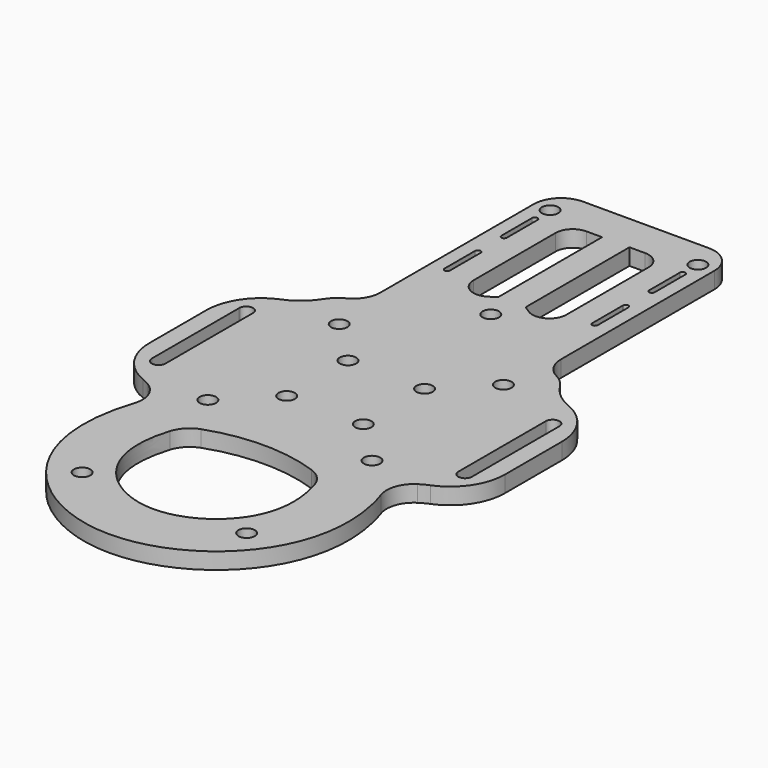
from build123d import *

# Parameters (mm, degrees)
F0_R     = 1.5
F1_DEPTH = 3


# Not quite as in the source:
# - ends of sketch curves that miss each other by under 0.0002 mm in the source are joined
# - the dataset's text gives a spline's control points without its knots; the knots are read off the source's solid
# - a feature names something its author has since deleted; it is built from what else it names


with BuildPart() as f1:
    # F0 (on Top) → F1 (new body)
    with BuildSketch(Plane.XY):
        with BuildLine():
            ThreePointArc((-16.5, 26.2979589711), (-17.2359856729, 23.6867941318), (-19.2272727273, 21.844341257))
            ThreePointArc((-19.2272727273, 21.844341257), (-20.5474988026, 20.9291933174), (-21.5775987425, 19.6965592455))
            ThreePointArc((-21.5775987425, 19.6965592455), (-23.6152839672, 17.3612838274), (-26.2701316567, 15.762078994))
            ThreePointArc((-26.2701316567, 15.762078994), (-30.7976296786, 12.0811595315), (-32.5, 6.5))
            Line((-32.5, 6.5), (-32.5, -6.5))
            ThreePointArc((-32.5, -6.5), (-30.7976296786, -12.0811595315), (-26.2701316567, -15.762078994))
            ThreePointArc((-26.2701316567, -15.762078994), (-25.4294357942, -16.1505865769), (-24.6282873533, -16.6152034628))
            ThreePointArc((-24.6282873533, -16.6152034628), (-22.6199096362, -19.1539208167), (-22.5875426225, -22.3908358966))
            add(Edge.make_bspline(
                [(-22.5875426225, -22.3908358966), (-29.1301810286, -42.1572830984), (0, -70.219824045), (29.1301810286, -42.1572830984), (22.5875426225, -22.3908358966)],
                knots=[0.0214687415, 0.0214687415, 0.0214687415, 0.0214687415, 0.5, 0.9785312585, 0.9785312585, 0.9785312585, 0.9785312585], degree=3))
            ThreePointArc((22.5875426225, -22.3908358966), (22.6199096362, -19.1539208167), (24.6282873533, -16.6152034628))
            ThreePointArc((24.6282873533, -16.6152034628), (25.4294357942, -16.1505865769), (26.2701316567, -15.762078994))
            ThreePointArc((26.2701316567, -15.762078994), (30.7976296786, -12.0811595315), (32.5, -6.5))
            Line((32.5, -6.5), (32.5, 6.5))
            ThreePointArc((32.5, 6.5), (30.7976296786, 12.0811595315), (26.2701316567, 15.762078994))
            ThreePointArc((26.2701316567, 15.762078994), (23.6152839672, 17.3612838274), (21.5775987425, 19.6965592455))
            ThreePointArc((21.5775987425, 19.6965592455), (20.5474988026, 20.9291933174), (19.2272727273, 21.844341257))
            ThreePointArc((19.2272727273, 21.844341257), (17.2359856729, 23.6867941318), (16.5, 26.2979589711))
            Line((16.5, 26.2979589711), (16.5, 61.2979589711))
            ThreePointArc((16.5, 61.2979589711), (15.0355339059, 64.8334928771), (11.5, 66.2979589711))
            Line((11.5, 66.2979589711), (-11.5, 66.2979589711))
            ThreePointArc((-11.5, 66.2979589711), (-15.0355339059, 64.8334928771), (-16.5, 61.2979589711))
            Line((-16.5, 61.2979589711), (-16.5, 26.2979589711))
        make_face()
        with Locations((-15.0325534991, -43.6784773437)):
            Circle(F0_R, mode=Mode.SUBTRACT)
        with Locations((-15, -15)):
            Circle(F0_R, mode=Mode.SUBTRACT)
        with Locations((-7, -7)):
            Circle(F0_R, mode=Mode.SUBTRACT)
        with Locations((15.0325534991, -43.6784773437)):
            Circle(F0_R, mode=Mode.SUBTRACT)
        with BuildLine():
            add(Edge.make_bspline(
                [(-13.2012257299, -25.8641514574), (-13.5472396089, -26.9597800065), (-14.1982208527, -29.7251957669), (-14.2899795625, -33.516748506), (-13.4270170307, -37.1167515894), (-11.7826738762, -40.1746977582), (-9.4323870949, -42.738127647), (-6.9985568447, -44.3715674999), (-4.8856018995, -45.3094299923), (-3.2540288337, -45.816960105), (-1.8857880841, -46.0707953295), (-0.8011676511, -46.1718209221), (0, -46.1969198965), (0.8011676511, -46.1718209221), (1.8857880841, -46.0707953295), (3.2540288337, -45.816960105), (4.8856018995, -45.3094299923), (6.9985568447, -44.3715674999), (9.4323870949, -42.738127647), (11.7826738762, -40.1746977582), (13.4270170307, -37.1167515894), (14.2899795625, -33.516748506), (14.1982208527, -29.7251957669), (13.5472396089, -26.9597800065), (13.2012257299, -25.8641514574)],
                knots=[0.0252083838, 0.0252083838, 0.0252083838, 0.0252083838, 0.0625, 0.125, 0.1875, 0.25, 0.3125, 0.375, 0.40625, 0.4375, 0.46875, 0.484375, 0.5, 0.515625, 0.53125, 0.5625, 0.59375, 0.625, 0.6875, 0.75, 0.8125, 0.875, 0.9375, 0.9747916162, 0.9747916162, 0.9747916162, 0.9747916162], degree=3))
            ThreePointArc((-13.2012257299, -25.8641514574), (-12.0290603688, -23.8957820907), (-10.1021030975, -22.656752593))
            ThreePointArc((-10.1021030975, -22.656752593), (0, -20.9211428123), (10.1021030975, -22.656752593))
            ThreePointArc((10.1021030975, -22.656752593), (12.0290603688, -23.8957820907), (13.2012257299, -25.8641514574))
        make_face(mode=Mode.SUBTRACT)
        with Locations((7, -7)):
            Circle(F0_R, mode=Mode.SUBTRACT)
        with Locations((15, -15)):
            Circle(F0_R, mode=Mode.SUBTRACT)
        with BuildLine():
            ThreePointArc((-29.2438267342, 10.1240768122), (-27.9378848559, 11.2484557296), (-26.75, 10))
            Line((-26.75, 10), (-26.75, -10))
            ThreePointArc((-26.75, -10), (-28.0001917269, -11.2499999853), (-29.2499999412, -9.9996165461))
            Line((-29.2499999412, -9.9996165461), (-29.2439026245, 9.8766863315))
            ThreePointArc((-29.2439026245, 9.8766863315), (-29.2499999412, 10.0003834539), (-29.2438267342, 10.1240768122))
        make_face(mode=Mode.SUBTRACT)
        with Locations((-15, 15)):
            Circle(F0_R, mode=Mode.SUBTRACT)
        with Locations((-7, 7)):
            Circle(F0_R, mode=Mode.SUBTRACT)
        with BuildLine():
            Line((-13.0075383335, 44.7114632656), (-13.0075383335, 37.8844546767))
            ThreePointArc((-13.0075383335, 37.8844546767), (-13, 37.7979589711), (-13.0075383335, 37.7114632656))
            ThreePointArc((-13.0075383335, 37.7114632656), (-13.5434117886, 37.2998471196), (-14, 37.7979589711))
            Line((-14, 37.7979589711), (-14, 44.7979589711))
            ThreePointArc((-14, 44.7979589711), (-13.5434117886, 45.2960708226), (-13.0075383335, 44.8844546767))
            ThreePointArc((-13.0075383335, 44.8844546767), (-13, 44.7979589711), (-13.0075383335, 44.7114632656))
        make_face(mode=Mode.SUBTRACT)
        with BuildLine():
            Line((-8.5, 37.5402642858), (-8.5, 56.2979589711))
            ThreePointArc((-8.5, 56.2979589711), (-7.5868990636, 58.5038831557), (-5.3818561331, 59.4191101782))
            Line((-5.3818561331, 59.4191101782), (-2.5, 59.4218882881))
            Line((-2.5, 59.4218882881), (-2.5, 35.7108392399))
            Line((-2.5, 35.7108392399), (-3.6436225473, 34.9459264474))
            ThreePointArc((-3.6436225473, 34.9459264474), (-6.8495091714, 34.7873117443), (-8.5, 37.5402642858))
        make_face(mode=Mode.SUBTRACT)
        with BuildLine():
            Line((-14, 50.7979589711), (-14, 57.7979589711))
            ThreePointArc((-14, 57.7979589711), (-13.5434117886, 58.2960708226), (-13.0075383335, 57.8844546767))
            ThreePointArc((-13.0075383335, 57.8844546767), (-13, 57.7979589711), (-13.0075383335, 57.7114632656))
            Line((-13.0075383335, 57.7114632656), (-13.0075383335, 50.8844546767))
            ThreePointArc((-13.0075383335, 50.8844546767), (-13, 50.7979589711), (-13.0075383335, 50.7114632656))
            ThreePointArc((-13.0075383335, 50.7114632656), (-13.5434117886, 50.2998471196), (-14, 50.7979589711))
        make_face(mode=Mode.SUBTRACT)
        with Locations((-13.5, 61.2979589711)):
            Circle(F0_R, mode=Mode.SUBTRACT)
        with Locations((7, 7)):
            Circle(F0_R, mode=Mode.SUBTRACT)
        with Locations((15, 15)):
            Circle(F0_R, mode=Mode.SUBTRACT)
        with Locations((0, 30.8675747365)):
            Circle(F0_R, mode=Mode.SUBTRACT)
        with BuildLine():
            ThreePointArc((29.2438267342, 10.1240768122), (29.2499999412, 10.0003834539), (29.2439026245, 9.8766863315))
            Line((29.2439026245, 9.8766863315), (29.2499999412, -9.9996165461))
            ThreePointArc((29.2499999412, -9.9996165461), (28.0001917269, -11.2499999853), (26.75, -10))
            Line((26.75, -10), (26.75, 10))
            ThreePointArc((26.75, 10), (27.9378848559, 11.2484557296), (29.2438267342, 10.1240768122))
        make_face(mode=Mode.SUBTRACT)
        with BuildLine():
            ThreePointArc((2.7271789356, 35.5588904396), (2.5603547361, 35.743081498), (2.5, 35.9841498812))
            Line((2.5, 35.9841498812), (2.5, 59.4218882881))
            Line((2.5, 59.4218882881), (5.3818561331, 59.4191101782))
            ThreePointArc((5.3818561331, 59.4191101782), (7.5868990636, 58.5038831557), (8.5, 56.2979589711))
            Line((8.5, 56.2979589711), (8.5, 37.5402642858))
            ThreePointArc((8.5, 37.5402642858), (6.8495091714, 34.7873117443), (3.6436225473, 34.9459264474))
            Line((3.6436225473, 34.9459264474), (2.7271789356, 35.5588904396))
        make_face(mode=Mode.SUBTRACT)
        with BuildLine():
            ThreePointArc((13.0075383335, 37.7114632656), (13, 37.7979589711), (13.0075383335, 37.8844546767))
            Line((13.0075383335, 37.8844546767), (13.0075383335, 44.7114632656))
            ThreePointArc((13.0075383335, 44.7114632656), (13, 44.7979589711), (13.0075383335, 44.8844546767))
            ThreePointArc((13.0075383335, 44.8844546767), (13.5434117886, 45.2960708226), (14, 44.7979589711))
            Line((14, 44.7979589711), (14, 37.7979589711))
            ThreePointArc((14, 37.7979589711), (13.5434117886, 37.2998471196), (13.0075383335, 37.7114632656))
        make_face(mode=Mode.SUBTRACT)
        with BuildLine():
            ThreePointArc((13.0075383335, 57.8844546767), (13.5434117886, 58.2960708226), (14, 57.7979589711))
            Line((14, 57.7979589711), (14, 50.7979589711))
            ThreePointArc((14, 50.7979589711), (13.5434117886, 50.2998471196), (13.0075383335, 50.7114632656))
            ThreePointArc((13.0075383335, 50.7114632656), (13, 50.7979589711), (13.0075383335, 50.8844546767))
            Line((13.0075383335, 50.8844546767), (13.0075383335, 57.7114632656))
            ThreePointArc((13.0075383335, 57.7114632656), (13, 57.7979589711), (13.0075383335, 57.8844546767))
        make_face(mode=Mode.SUBTRACT)
        with Locations((13.5, 61.2979589711)):
            Circle(F0_R, mode=Mode.SUBTRACT)
    extrude(amount=F1_DEPTH)


solid = f1.part
